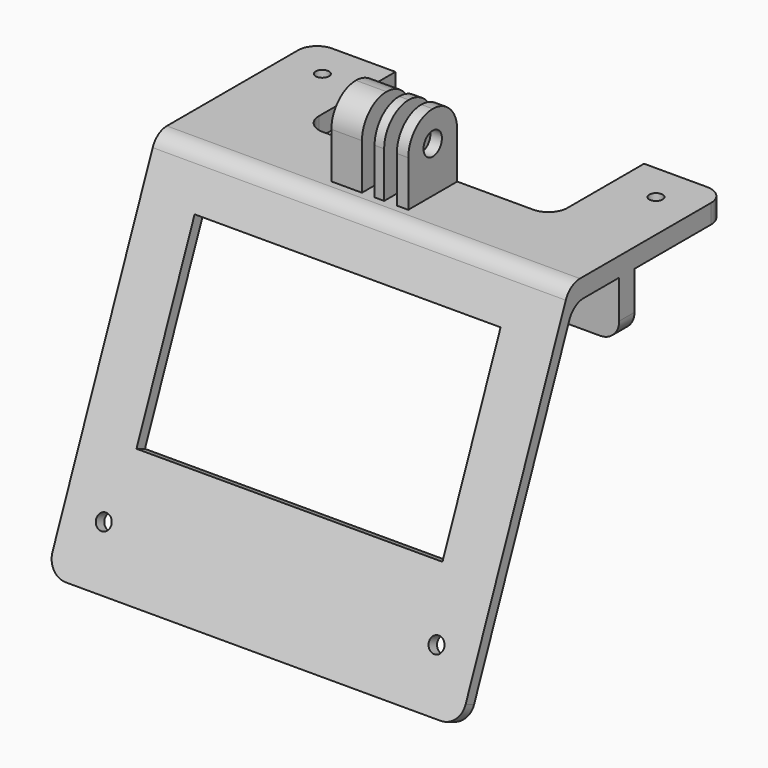
from build123d import *

# Parameters (mm, degrees)
F0_W      = 21.5
F0_H      = 30
F1_DEPTH  = 5
F3_DEPTH  = 108
F4_R      = 2
F5_DEPTH  = 25
F7_R      = 5
F6_W      = 8
F6_H      = 16
F6_W_2    = 2.5
F6_W_3    = 3
F8_DEPTH  = 20
F9_R      = 7.99999
F10_R     = 3
F11_DEPTH = 40
F12_W     = 80
F12_H     = 50
F13_DEPTH = 25
F15_DEPTH = 15
F16_R     = 5
F17_R     = 1.75
F18_DEPTH = 25


# Not quite as in the source:
# - a fillet or chamfer is up to 0.001 mm smaller than in the source, because OpenCascade refuses the exact size


with BuildPart() as f1:
    # F0 (on Top) → F1 (new body)
    with BuildSketch(Plane.XY):
        with Locations((-43.25, 15)):
            Rectangle(F0_W, F0_H)
        Polygon((-32.5, 0), (-54, 0), (-54, -20), (54, -20), (54, 0), (32.5, 0), align=None)
        with Locations((43.25, 15)):
            Rectangle(F0_W, F0_H)
    extrude(amount=F1_DEPTH)

    # F2 (on face) → F3 (join)
    with BuildSketch(Plane(origin=(-54, 0, 0), x_dir=(0, -1, 0), z_dir=(-1, 0, 0))):
        Polygon((20, 5), (20, 0), (54.3258497444, -83.6021589144), (57.101034605, -82.4627077355), (21.1900987758, 5), align=None)
    extrude(amount=-F3_DEPTH)

    # F4 (on face) → F5 (cut)
    with BuildSketch(Plane(origin=(0, -19.8899648845, 8.1665348708), x_dir=(1, 0, 0), z_dir=(0, -0.9250616202, 0.3798170597))):
        with Locations((-43.5, -83.4230529098)):
            Circle(F4_R)
        with Locations((43.5, -83.4230529098)):
            Circle(F4_R)
    extrude(amount=-F5_DEPTH, mode=Mode.SUBTRACT)

    # F7
    f7_edges = [f1.edges().sort_by_distance(p)[0] for p in [
        (0, -21.190099, 5),
        (0, -20, 0),
        (-54, 30, 2.5),
        (54, 30, 2.5),
        (54, -55.713442, -83.032433),
        (-54, -55.713442, -83.032433),
        (-32.5, 0, 2.5),
        (32.5, 0, 2.5),
    ]]
    fillet(f7_edges, radius=F7_R)

    # F6 (on face) → F8 (join)
    with BuildSketch(Plane.XY.offset(5)):
        with Locations((-8.45, -8)):
            Rectangle(F6_W, F6_H)
        with Locations((0.1, -8)):
            Rectangle(F6_W_2, F6_H)
        with Locations((6.15, -8)):
            Rectangle(F6_W_3, F6_H)
    extrude(amount=F8_DEPTH)

    # F9 (radius 8 in the source; OpenCascade refuses exactly that, so slightly less here)
    f9_edges = [f1.edges().sort_by_distance(p)[0] for p in [
        (-8.45, -16, 25),
        (0.1, -16, 25),
        (6.15, -16, 25),
        (-8.45, 0, 25),
        (0.1, 0, 25),
        (6.15, 0, 25),
    ]]
    fillet(f9_edges, radius=F9_R)

    # F10 (on face) → F11 (cut)
    with BuildSketch(Plane.YZ.offset(7.65)):
        with Locations((-8, 17)):
            Circle(F10_R)
    extrude(amount=-F11_DEPTH, mode=Mode.SUBTRACT)

    # F12 (on face) → F13 (cut)
    with BuildSketch(Plane(origin=(0, -19.8899648845, 8.1665348708), x_dir=(1, 0, 0), z_dir=(0, -0.9250616202, 0.3798170597))):
        with Locations((0, -41.7751698217)):
            Rectangle(F12_W, F12_H)
    extrude(amount=-F13_DEPTH, mode=Mode.SUBTRACT)

    # F14 (on face) → F15 (join)
    with BuildSketch(Plane(origin=(0, 0, 0), x_dir=(1, 0, 0), z_dir=(0, 0, -1))):
        Polygon((-54, 5), (-54, 0), (-27.5, 0), (27.5, 0), (54, 0), (54, 5), align=None)
    extrude(amount=F15_DEPTH)

    # F16
    f16_edges = [f1.edges().sort_by_distance(p)[0] for p in [
        (54, -2.5, -15),
        (-54, -2.5, -15),
    ]]
    fillet(f16_edges, radius=F16_R)

    # F17 (on face) → F18 (cut)
    with BuildSketch(Plane.XY.offset(5)):
        with Locations((-43.6119101942, 20)):
            Circle(F17_R)
        with Locations((43.6119101942, 20)):
            Circle(F17_R)
    extrude(amount=-F18_DEPTH, mode=Mode.SUBTRACT)


solid = f1.part
